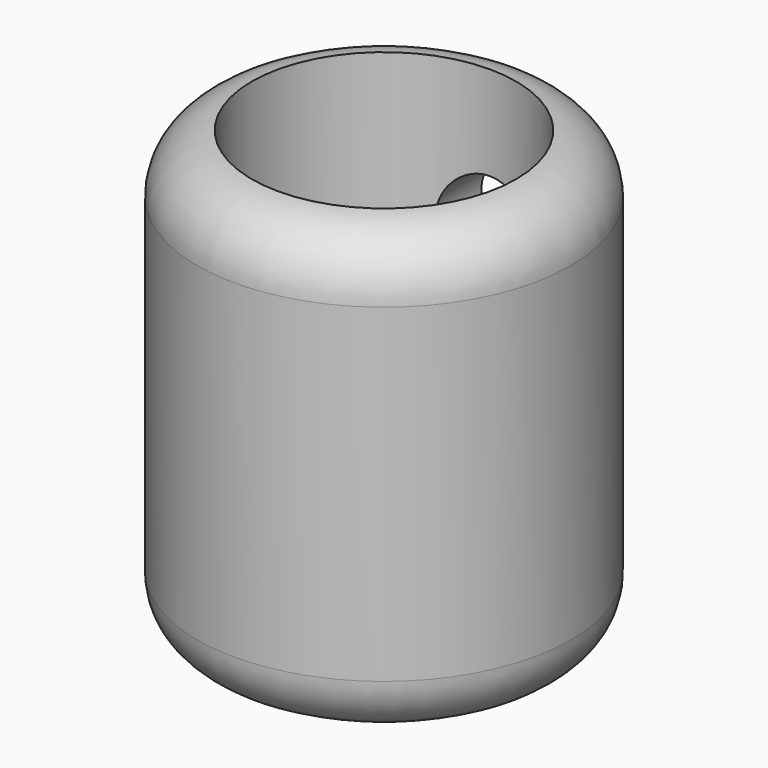
from build123d import *

# Parameters (mm, degrees)
F0_R     = 15.875
F0_R_2   = 11.25
F1_DEPTH = 38
F3_R     = 4
F4_DEPTH = 15.876


# Not quite as in the source:
# - a fillet or chamfer that OpenCascade refuses, or shapes differently, is made with other operations: its cross-section is extruded or revolved along the edge and cut away or added


with BuildPart() as f1:
    # F0 (on Top) → F1 (new body)
    with BuildSketch(Plane.XY):
        Circle(F0_R)
        Circle(F0_R_2, mode=Mode.SUBTRACT)
    extrude(amount=F1_DEPTH)

    # F2: fillet of radius 5 on 2 edges, made by hand

    # F2_s1 → F2_t2 (revolve, cut)
    with BuildSketch(Plane.XZ):
        with BuildLine():
            ThreePointArc((15.875, 33.0140823312), (14.5407195747, 36.4144499584), (11.25, 38))
            Line((11.25, 38), (15.875, 38))
            Line((15.875, 38), (15.875, 33.0140823312))
        make_face()
    revolve(axis=Axis((0, 0, 38), (0, 0, 1)), mode=Mode.SUBTRACT)

    # F2_s3 → F2_t4 (revolve, cut)
    with BuildSketch(Plane.XZ):
        with BuildLine():
            ThreePointArc((15.875, 4.9859176688), (14.5407195747, 1.5855500416), (11.25, 0))
            Line((11.25, 0), (15.875, 0))
            Line((15.875, 0), (15.875, 4.9859176688))
        make_face()
    revolve(axis=Axis((0, 0, 0), (0, 0, 1)), mode=Mode.SUBTRACT)

    # F3 (on Front) → F4 (cut, through all)
    with BuildSketch(Plane.XZ):
        with Locations((0, 12)):
            Circle(F3_R)
        with Locations((0, 26)):
            Circle(F3_R)
    extrude(amount=-F4_DEPTH, mode=Mode.SUBTRACT)


solid = f1.part
